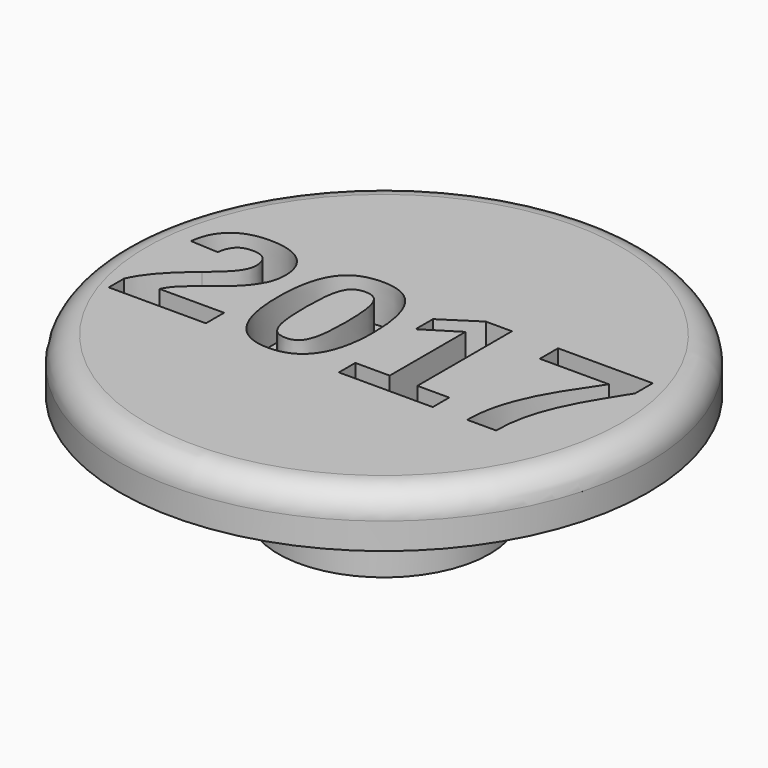
from build123d import *

# Parameters (mm, degrees)
F0_R         = 4
F1_DEPTH     = 6
F0_R_2       = 5
F2_DEPTH     = 2.5
F0_R_3       = 10
F3_DEPTH     = 2
F4_R         = 1
F5_TEXT_SIZE = 7.6388888889
F6_DEPTH     = 1.5


# Not quite as in the source:
# - Text() gives the source's letters only with a copy of the font that has no kerning and outlines rounded to 1/6400 em; it was checked with that copy


with BuildPart() as f1:
    # F0 (on Top) → F1 (new body)
    with BuildSketch(Plane.XY):
        Circle(F0_R)
    extrude(amount=-F1_DEPTH)

    # F0 (on Top) → F2 (join)
    with BuildSketch(Plane.XY):
        Circle(F0_R_2)
        Circle(F0_R, mode=Mode.SUBTRACT)
    extrude(amount=-F2_DEPTH)

    # F0 (on Top) → F3 (join)
    with BuildSketch(Plane.XY):
        Circle(F0_R_3)
        Circle(F0_R_2, mode=Mode.SUBTRACT)
    extrude(amount=-F3_DEPTH)

    # F4
    f4_edges = [f1.edges().sort_by_distance(p)[0] for p in [
        (-10, 0, 0),
    ]]
    fillet(f4_edges, radius=F4_R)

    # F5 (on Top) → F6 (cut)
    with BuildSketch(Plane.XY):
        with Locations((-8.5221575535, -2.7051233415)):
            Text('2017', F5_TEXT_SIZE, font='Arimo', font_style=FontStyle.BOLD, text_align=(TextAlign.LEFT, TextAlign.BOTTOM))
    extrude(amount=-F6_DEPTH, mode=Mode.SUBTRACT)


solid = f1.part
